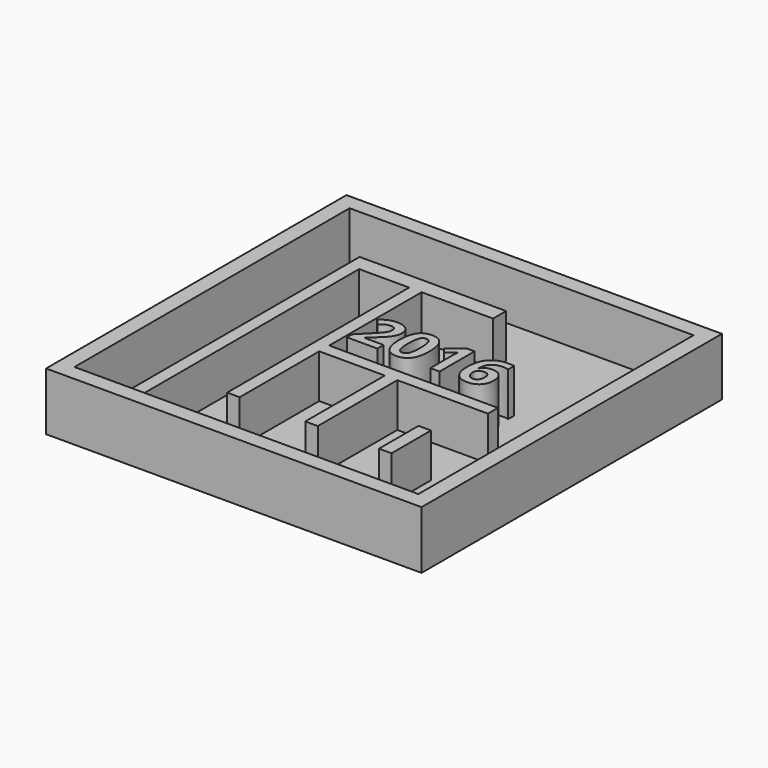
from build123d import *

# Parameters (mm, degrees)
F0_W         = 38.1
F0_H         = 38.1
F1_DEPTH     = 0.79375
F2_W         = 38.1
F2_H         = 38.1
F2_W_2       = 34.8996
F2_H_2       = 34.8996
F3_DEPTH     = 5.08
F5_DEPTH     = 4.445
F6_R         = 1.27
F7_DEPTH     = 0.396875
F4_W         = 1.27
F4_H         = 5.009116171
F4_TEXT_SIZE = 6.210664934
F8_DEPTH     = 4.445
F9_DEPTH     = 4.445
F10_DEPTH    = 4.445


# Not quite as in the source:
# - Text() gives the source's letters only with a copy of the font that has no kerning and outlines rounded to 1/6400 em; it was checked with that copy


with BuildPart() as f1:
    # F0 (on Top) → F1 (new body)
    with BuildSketch(Plane.XY):
        with Locations((4.7945361584, -11.7150577805)):
            Rectangle(F0_W, F0_H)
    extrude(amount=F1_DEPTH)

    # F2 (on face) → F3 (join)
    with BuildSketch(Plane.XY.offset(0.79375)):
        with Locations((4.7945361584, -11.7150577805)):
            Rectangle(F2_W, F2_H)
        with Locations((4.7945361584, -11.7150577805)):
            Rectangle(F2_W_2, F2_H_2, mode=Mode.SUBTRACT)
    extrude(amount=F3_DEPTH)

    # F4 (on face) → F5 (join)
    with BuildSketch(Plane.XY.offset(0.79375)):
        Polygon((-7.5752638416, 0.6547422195), (-7.5752638416, -29.1648577805), (-6.3052638416, -29.1648577805), (-6.3052638416, -1.0010383929), (-6.3052638416, 0.6547422195), align=None)
    extrude(amount=F5_DEPTH)

    # F6 (on face) → F7 (cut)
    with BuildSketch(Plane.XY.offset(0.79375)):
        with Locations((-10.4948775843, -24.9380301684)):
            Circle(F6_R)
        with Locations((-3.5624078009, -4.247973673)):
            Circle(F6_R)
    extrude(amount=-F7_DEPTH, mode=Mode.SUBTRACT)

    # F4 (on face) → F8 (join)
    with BuildSketch(Plane.XY.offset(0.79375)):
        Polygon((-7.5752638416, 0.6547422195), (-7.5752638416, -29.1648577805), (-6.3052638416, -29.1648577805), (-6.3052638416, -1.0010383929), (-6.3052638416, 0.6547422195), align=None)
        Polygon((-6.3052638416, 0.6547422195), (-6.3052638416, -1.0010383929), (-1.2252638416, -1.0010383929), (0.0447361584, -1.0010383929), (7.2880764492, -1.0010383929), (7.2880764492, 0.6547422195), (3.6642965861, 0.6547422195), (-1.2252638416, 0.6547422195), align=None)
        Polygon((0.0447361584, -1.0010383929), (-1.2252638416, -1.0010383929), (-1.2252638416, -1.3666254385), (-1.2252638416, -12.7257416095), (-1.2252638416, -13.9957416095), (-1.2252638416, -24.0848577805), (0.0447361584, -24.0848577805), (0.0447361584, -13.9957416095), (6.6995361584, -13.9957416095), (6.6995361584, -24.0848577805), (7.9695361584, -24.0848577805), (7.9695361584, -13.9957416095), (17.1643361584, -13.9957416095), (17.1643361584, -12.7257416095), (7.9695361584, -12.7257416095), (5.6569511071, -12.7257416095), (0.0447361584, -12.7257416095), align=None)
        with Locations((14.8128645802, -21.580299695)):
            Rectangle(F4_W, F4_H)
        with Locations((0.0038469443, -10.7453092933)):
            Text('2016', F4_TEXT_SIZE, font='Open Sans', font_style=FontStyle.BOLD, text_align=(TextAlign.LEFT, TextAlign.BOTTOM))
    extrude(amount=F8_DEPTH)

    # F4 (on face) → F9 (join)
    with BuildSketch(Plane.XY.offset(0.79375)):
        Polygon((-7.5752638416, 0.6547422195), (-7.5752638416, -29.1648577805), (-6.3052638416, -29.1648577805), (-6.3052638416, -1.0010383929), (-6.3052638416, 0.6547422195), align=None)
        Polygon((-6.3052638416, 0.6547422195), (-6.3052638416, -1.0010383929), (-1.2252638416, -1.0010383929), (0.0447361584, -1.0010383929), (7.2880764492, -1.0010383929), (7.2880764492, 0.6547422195), (3.6642965861, 0.6547422195), (-1.2252638416, 0.6547422195), align=None)
        Polygon((0.0447361584, -1.0010383929), (-1.2252638416, -1.0010383929), (-1.2252638416, -1.3666254385), (-1.2252638416, -12.7257416095), (-1.2252638416, -13.9957416095), (-1.2252638416, -24.0848577805), (0.0447361584, -24.0848577805), (0.0447361584, -13.9957416095), (6.6995361584, -13.9957416095), (6.6995361584, -24.0848577805), (7.9695361584, -24.0848577805), (7.9695361584, -13.9957416095), (17.1643361584, -13.9957416095), (17.1643361584, -12.7257416095), (7.9695361584, -12.7257416095), (5.6569511071, -12.7257416095), (0.0447361584, -12.7257416095), align=None)
        with Locations((14.8128645802, -21.580299695)):
            Rectangle(F4_W, F4_H)
        with Locations((0.0038469443, -10.7453092933)):
            Text('2016', F4_TEXT_SIZE, font='Open Sans', font_style=FontStyle.BOLD, text_align=(TextAlign.LEFT, TextAlign.BOTTOM))
    extrude(amount=F9_DEPTH)

    # F4 (on face) → F10 (join)
    with BuildSketch(Plane.XY.offset(0.79375)):
        Polygon((-7.5752638416, 0.6547422195), (-7.5752638416, -29.1648577805), (-6.3052638416, -29.1648577805), (-6.3052638416, -1.0010383929), (-6.3052638416, 0.6547422195), align=None)
        Polygon((-6.3052638416, 0.6547422195), (-6.3052638416, -1.0010383929), (-1.2252638416, -1.0010383929), (0.0447361584, -1.0010383929), (7.2880764492, -1.0010383929), (7.2880764492, 0.6547422195), (3.6642965861, 0.6547422195), (-1.2252638416, 0.6547422195), align=None)
        Polygon((0.0447361584, -1.0010383929), (-1.2252638416, -1.0010383929), (-1.2252638416, -1.3666254385), (-1.2252638416, -12.7257416095), (-1.2252638416, -13.9957416095), (-1.2252638416, -24.0848577805), (0.0447361584, -24.0848577805), (0.0447361584, -13.9957416095), (6.6995361584, -13.9957416095), (6.6995361584, -24.0848577805), (7.9695361584, -24.0848577805), (7.9695361584, -13.9957416095), (17.1643361584, -13.9957416095), (17.1643361584, -12.7257416095), (7.9695361584, -12.7257416095), (5.6569511071, -12.7257416095), (0.0447361584, -12.7257416095), align=None)
        with Locations((14.8128645802, -21.580299695)):
            Rectangle(F4_W, F4_H)
        with Locations((0.0038469443, -10.7453092933)):
            Text('2016', F4_TEXT_SIZE, font='Open Sans', font_style=FontStyle.BOLD, text_align=(TextAlign.LEFT, TextAlign.BOTTOM))
    extrude(amount=F10_DEPTH)


solid = f1.part
